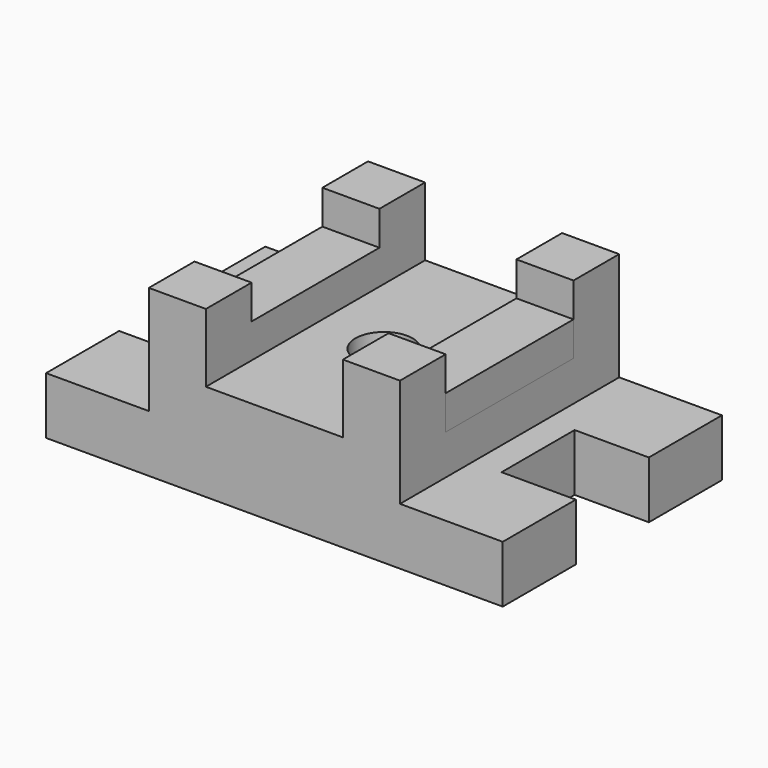
from build123d import *

# Parameters (mm, degrees)
F1_DEPTH = 15.875
F2_W     = 69.85
F2_H     = 76.2
F2_R     = 7.9375
F3_DEPTH = 11.1125
F4_DEPTH = 15.876
F5_W     = 15.875
F5_H     = 15.875
F6_DEPTH = 19.05
F7_W     = 15.875
F7_H     = 44.45
F8_DEPTH = 9.525


# Not quite as in the source:
# - a length typed as a fraction of an inch, garbled in the dataset ("3 / 203.2 mm" for 3/8 in), is restored


with BuildPart() as f1:
    # F0 (on Top) → F1 (new body)
    with BuildSketch(Plane.XY):
        Polygon((63.5, 12.7), (63.5, 38.1), (-63.5, 38.1), (-63.5, 12.7), (-42.8498, 12.7), (-42.8498, -12.7), (-63.5, -12.7), (-63.5, -38.1), (63.5, -38.1), (63.5, -12.7), (42.8498, -12.7), (42.8498, 12.7), align=None)
    extrude(amount=F1_DEPTH)

    # F2 (on face) → F3 (join)
    with BuildSketch(Plane.XY.offset(15.875)):
        Rectangle(F2_W, F2_H)
        Circle(F2_R, mode=Mode.SUBTRACT)
    extrude(amount=F3_DEPTH)

    # F4 (cut, through all): a face of the model
    f4_faces = [f1.faces().sort_by_distance(p)[0] for p in [
        (0, 0, 15.875),
    ]]
    extrude(f4_faces, amount=-F4_DEPTH, mode=Mode.SUBTRACT)

    # F5 (on face) → F6 (join)
    with BuildSketch(Plane.XY.offset(26.9875)):
        with Locations((-26.9875, 30.1625)):
            Rectangle(F5_W, F5_H)
        with Locations((26.9875, 30.1625)):
            Rectangle(F5_W, F5_H)
        with Locations((26.9875, -30.1625)):
            Rectangle(F5_W, F5_H)
        with Locations((-26.9875, -30.1625)):
            Rectangle(F5_W, F5_H)
    extrude(amount=F6_DEPTH)

    # F7 (on face) → F8 (join)
    with BuildSketch(Plane.XY.offset(26.9875)):
        with Locations((26.9875, 0)):
            Rectangle(F7_W, F7_H)
        with Locations((-26.9875, 0)):
            Rectangle(F7_W, F7_H)
    extrude(amount=F8_DEPTH)


solid = f1.part
